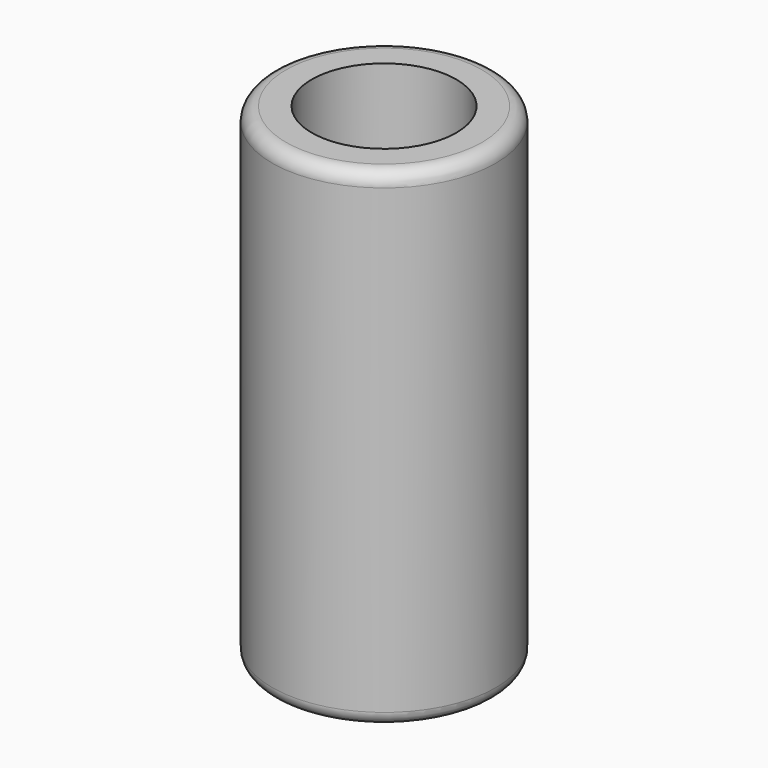
from build123d import *

# Parameters (mm, degrees)
F0_R     = 25.3953088791
F1_DEPTH = 111
F2_T     = -9
F3_R     = 3.1384776311


with BuildPart() as f1:
    # F0 (on Top) → F1 (new body)
    with BuildSketch(Plane.XY):
        Circle(F0_R)
    extrude(amount=F1_DEPTH)

    # F2
    f2_openings = [f1.faces().sort_by_distance(p)[0] for p in [
        (0, 0, 111),
    ]]
    offset(amount=F2_T, openings=f2_openings)

    # F3
    f3_edges = [f1.edges().sort_by_distance(p)[0] for p in [
        (25.395309, 0, 55.5),
        (-25.395309, 0, 0),
        (-25.395309, 0, 111),
        (-16.395309, 0, 9),
    ]]
    fillet(f3_edges, radius=F3_R)


solid = f1.part
